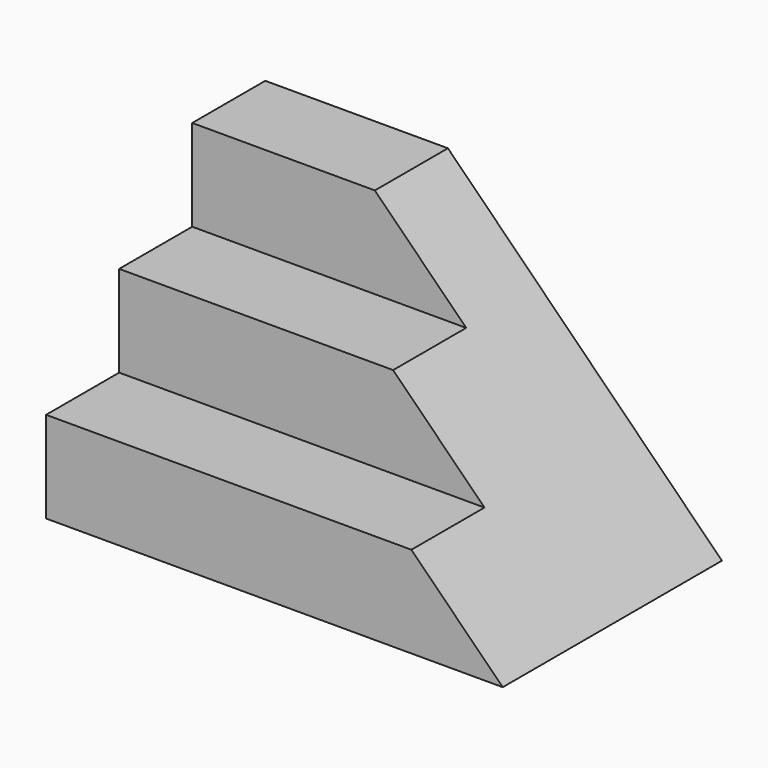
from build123d import *

# Parameters (mm, degrees)
F1_DEPTH = 100
F2_SIZE2 = 59.99999
F2_SIZE  = 59.99999


# Not quite as in the source:
# - a fillet or chamfer is up to 0.001 mm smaller than in the source, because OpenCascade refuses the exact size


with BuildPart() as f1:
    # F0 (on Right) → F1 (new body)
    with BuildSketch(Plane.YZ):
        Polygon((-60, 0), (0, 0), (0, 60), (-20, 60), (-20, 40), (-40, 40), (-40, 20), (-60, 20), align=None)
    extrude(amount=F1_DEPTH)

    # F2 (size 60 and 60 in the source; OpenCascade refuses exactly that, so slightly less here)
    f2_edges = [f1.edges().sort_by_distance(p)[0] for p in [
        (100, -10, 60),
    ]]
    chamfer(f2_edges, length=F2_SIZE, length2=F2_SIZE2)


solid = f1.part
